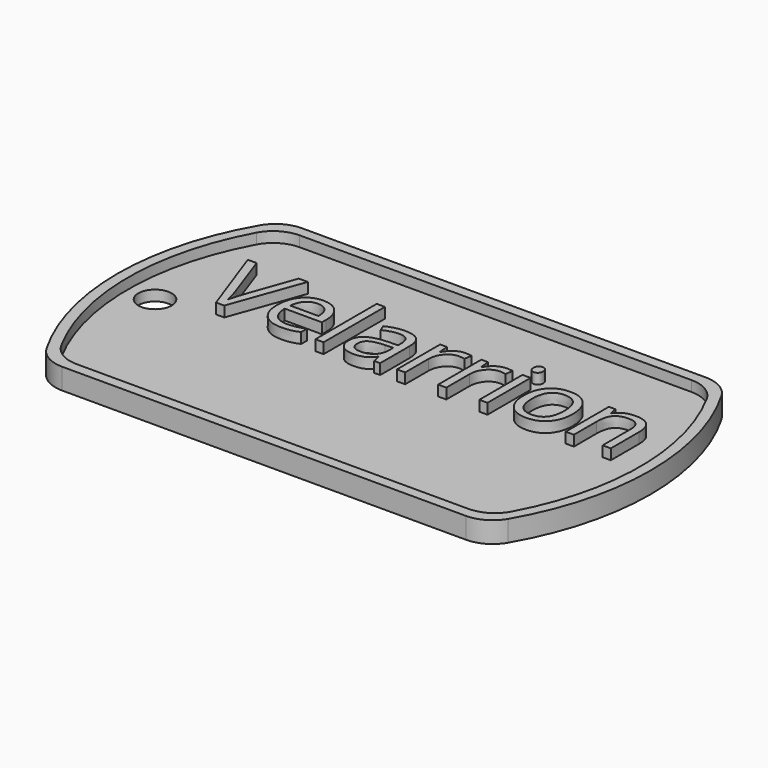
from build123d import *

# Parameters (mm, degrees)
F1_DEPTH     = 1
F3_DEPTH     = 1
F4_R         = 1.5875
F5_DEPTH     = 1
F6_TEXT_SIZE = 9.6068611634
F7_DEPTH     = 1
F8_DEPTH     = 1


# Not quite as in the source:
# - Text() gives the source's letters only with a copy of the font that has no kerning and outlines rounded to 1/6400 em; it was checked with that copy


with BuildPart() as f1:
    # F0 (on Top) → F1 (new body)
    with BuildSketch(Plane.XY):
        with BuildLine():
            ThreePointArc((-19.2474145991, 14.2875), (-20.8349145991, 13.862130657), (-21.9970452561, 12.7))
            ThreePointArc((-21.9970452561, 12.7), (-25.4, 0), (-21.9970452561, -12.7))
            ThreePointArc((-21.9970452561, -12.7), (-20.8349145991, -13.862130657), (-19.2474145991, -14.2875))
            Line((-19.2474145991, -14.2875), (19.2474145991, -14.2875))
            ThreePointArc((19.2474145991, -14.2875), (20.8349145991, -13.862130657), (21.9970452561, -12.7))
            ThreePointArc((21.9970452561, -12.7), (25.4, 0), (21.9970452561, 12.7))
            ThreePointArc((21.9970452561, 12.7), (20.8349145991, 13.862130657), (19.2474145991, 14.2875))
            Line((19.2474145991, 14.2875), (-19.2474145991, 14.2875))
        make_face()
    extrude(amount=F1_DEPTH)

    # F2 (on face) → F3 (join)
    with BuildSketch(Plane.XY.offset(1)):
        with BuildLine():
            Line((19.2474145991, 14.2875), (-19.2474145991, 14.2875))
            ThreePointArc((-19.2474145991, 14.2875), (-20.8349145991, 13.862130657), (-21.9970452561, 12.7))
            ThreePointArc((-21.9970452561, 12.7), (-25.4, 0), (-21.9970452561, -12.7))
            ThreePointArc((-21.9970452561, -12.7), (-20.8349145991, -13.862130657), (-19.2474145991, -14.2875))
            Line((-19.2474145991, -14.2875), (19.2474145991, -14.2875))
            ThreePointArc((19.2474145991, -14.2875), (20.8349145991, -13.862130657), (21.9970452561, -12.7))
            ThreePointArc((21.9970452561, -12.7), (25.4, 0), (21.9970452561, 12.7))
            ThreePointArc((21.9970452561, 12.7), (20.8349145991, 13.862130657), (19.2474145991, 14.2875))
        make_face()
        with BuildLine():
            ThreePointArc((-21.4526124879, 11.6252061249), (-20.2856017842, 12.8404540819), (-18.6611352482, 13.2875))
            Line((-18.6611352482, 13.2875), (18.6611352482, 13.2875))
            ThreePointArc((18.6611352482, 13.2875), (20.2856017842, 12.8404540819), (21.4526124879, 11.6252061249))
            ThreePointArc((21.4526124879, 11.6252061249), (24.4, 0), (21.4526124879, -11.6252061249))
            ThreePointArc((21.4526124879, -11.6252061249), (20.2856017842, -12.8404540819), (18.6611352482, -13.2875))
            Line((18.6611352482, -13.2875), (-18.6611352482, -13.2875))
            ThreePointArc((-18.6611352482, -13.2875), (-20.2856017842, -12.8404540819), (-21.4526124879, -11.6252061249))
            ThreePointArc((-21.4526124879, -11.6252061249), (-24.4, 0), (-21.4526124879, 11.6252061249))
        make_face(mode=Mode.SUBTRACT)
    extrude(amount=F3_DEPTH)

    # F4 (on face) → F5 (cut)
    with BuildSketch(Plane.XY.offset(1)):
        with Locations((-21.821282804, 0)):
            Circle(F4_R)
    extrude(amount=-F5_DEPTH, mode=Mode.SUBTRACT)

    # F6 (on face) → F7 (join)
    with BuildSketch(Plane.XY.offset(1)):
        with Locations((-19.2244183272, 0.9450849029)):
            Text('Velarrion', F6_TEXT_SIZE, font='Open Sans', text_align=(TextAlign.LEFT, TextAlign.BOTTOM))
    extrude(amount=F7_DEPTH)

    # F6 (on face) → F8 (join)
    with BuildSketch(Plane.XY.offset(1)):
        with Locations((-19.2244183272, 0.9450849029)):
            Text('Velarrion', F6_TEXT_SIZE, font='Open Sans', text_align=(TextAlign.LEFT, TextAlign.BOTTOM))
    extrude(amount=F8_DEPTH)


solid = f1.part
